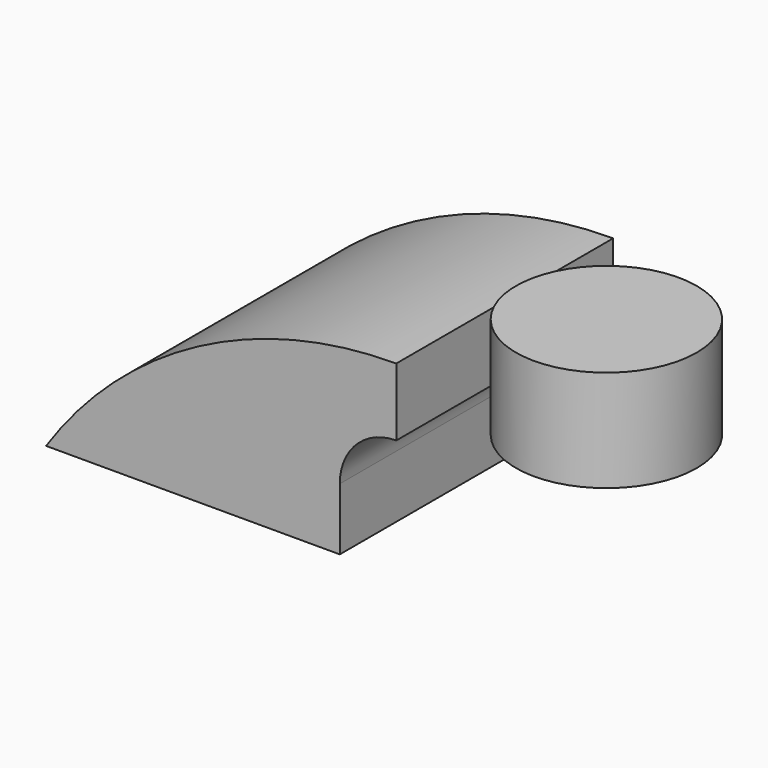
from build123d import *

# Parameters (mm, degrees)
F2_DEPTH = 38.1


# Not quite as in the source:
# - the program builds the solid bodies; features that only make, move or delete a surface that nothing else refers to are left out


with BuildPart() as f2:
    # F0 (on Front) → F2 (new body, symmetric)
    with BuildSketch(Plane.XZ):
        with BuildLine():
            Line((22.225, 9.525), (41.275, 9.525))
            Line((41.275, 9.525), (41.275, 27.0002))
            ThreePointArc((41.275, 27.0002), (45.9246798487, 38.2255201513), (57.15, 42.8752))
            Line((57.15, 42.8752), (57.15, 61.9252))
            ThreePointArc((57.15, 61.9252), (32.4542956671, 51.6959043329), (22.225, 27.0002))
            Line((22.225, 27.0002), (22.225, 9.525))
        make_face()
        with BuildLine():
            ThreePointArc((57.15, 61.9252), (1.3977319182, 48.0089590969), (-41.275, 9.525))
            Line((-41.275, 9.525), (22.225, 9.525))
            Line((22.225, 9.525), (22.225, 27.0002))
            ThreePointArc((22.225, 27.0002), (32.4542956671, 51.6959043329), (57.15, 61.9252))
        make_face()
    extrude(amount=F2_DEPTH, both=True)


with BuildPart() as f3:
    # F0 (on Front) → F3 (revolve)
    with BuildSketch(Plane.XZ):
        Polygon((85.725, 66.675), (85.725, 61.9252), (85.725, 52.3875), (85.725, 42.8752), (85.725, 38.1), (111.125, 38.1), (111.125, 66.675), align=None)
    revolve(axis=Axis((85.725, 0, 50.0126), (0, 0, 1)))


solid = Compound([f2.part, f3.part])
